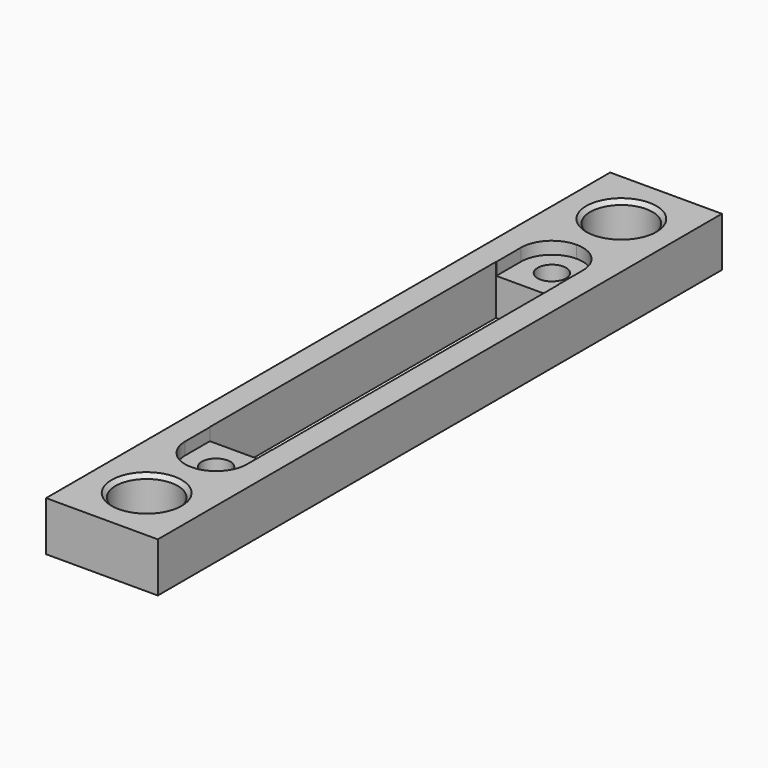
from build123d import *

# Parameters (mm, degrees)
F0_W     = 14.35
F0_H     = 90.5499906
F0_R     = 4
F0_R_2   = 1.8288
F0_W_2   = 8
F0_H_2   = 45.9749906
F1_DEPTH = 6.35
F2_SIZE  = 0.254
F3_W     = 7.9375
F3_H     = 7.9375
F4_DEPTH = 1.5875
F5_R     = 3.96874
F6_SIZE  = 0.508


# Not quite as in the source:
# - a fillet or chamfer is up to 0.001 mm smaller than in the source, because OpenCascade refuses the exact size


with BuildPart() as f1:
    # F0 (on Top) → F1 (new body)
    with BuildSketch(Plane.XY):
        Rectangle(F0_W, F0_H)
        with Locations((0, -38.0999953)):
            Circle(F0_R, mode=Mode.SUBTRACT)
        with Locations((0, -26.9562453)):
            Circle(F0_R_2, mode=Mode.SUBTRACT)
        Rectangle(F0_W_2, F0_H_2, mode=Mode.SUBTRACT)
        with Locations((0, 26.9562453)):
            Circle(F0_R_2, mode=Mode.SUBTRACT)
        with Locations((0, 38.0999953)):
            Circle(F0_R, mode=Mode.SUBTRACT)
    extrude(amount=F1_DEPTH)

    # F2
    f2_edges = [f1.edges().sort_by_distance(p)[0] for p in [
        (-4, 38.099995, 0),
        (-4, -38.099995, 0),
    ]]
    chamfer(f2_edges, length=F2_SIZE)

    # F3 (on face) → F4 (cut)
    with BuildSketch(Plane.XY.offset(6.35)):
        with Locations((0, 26.9562453)):
            Rectangle(F3_W, F3_H)
        with Locations((0, -26.9562453)):
            Rectangle(F3_W, F3_H)
    extrude(amount=-F4_DEPTH, mode=Mode.SUBTRACT)

    # F5 (radius 3.96875 in the source; OpenCascade refuses exactly that, so slightly less here)
    f5_edges = [f1.edges().sort_by_distance(p)[0] for p in [
        (-3.96875, -30.924995, 5.55625),
        (3.96875, -30.924995, 5.55625),
        (-3.96875, 30.924995, 5.55625),
        (3.96875, 30.924995, 5.55625),
    ]]
    fillet(f5_edges, radius=F5_R)

    # F6
    f6_edges = [f1.edges().sort_by_distance(p)[0] for p in [
        (-4, 38.099995, 6.35),
        (-4, -38.099995, 6.35),
    ]]
    chamfer(f6_edges, length=F6_SIZE)


solid = f1.part
